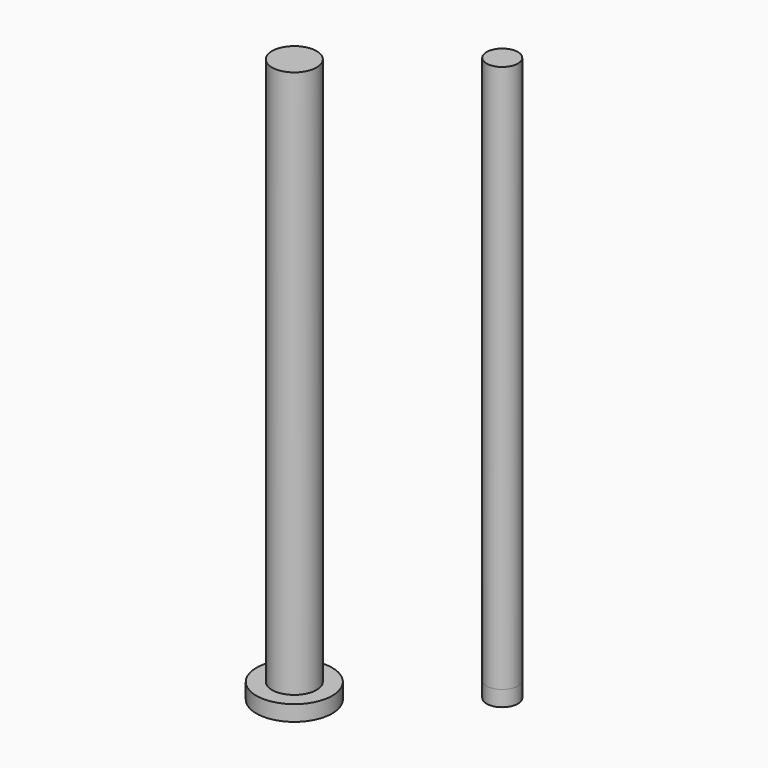
from build123d import *

# Parameters (mm, degrees)
F0_R      = 2.85
F1_DEPTH  = 70.1
F0_R_2    = 2
F0_R_3    = 4.85
F1_FACE_R = 2.85
F2_DEPTH  = 2


with BuildPart() as f1:
    # F0 (on Top) → F1 (new body)
    with BuildSketch(Plane.XY):
        Circle(F0_R)
    extrude(amount=F1_DEPTH)

    # F0 (on Top) + F1_face (on face) → F2 (join)
    with BuildSketch(Plane.XY):
        Circle(F0_R_3)
        Circle(F0_R, mode=Mode.SUBTRACT)
        with Locations((16.0180740058, 13.2293421775)):
            Circle(F0_R_2)
    with BuildSketch(Plane(origin=(0, 0, 0), x_dir=(1, 0, 0), z_dir=(0, 0, -1))):
        Circle(F1_FACE_R)
    extrude(amount=-F2_DEPTH, dir=(0, 0, 1))


with BuildPart() as f1b:
    # F0 (on Top) → F1, piece 2 (new body)
    with BuildSketch(Plane.XY):
        with Locations((16.0180740058, 13.2293421775)):
            Circle(F0_R_2)
    extrude(amount=F1_DEPTH)


solid = Compound([f1.part, f1b.part])
